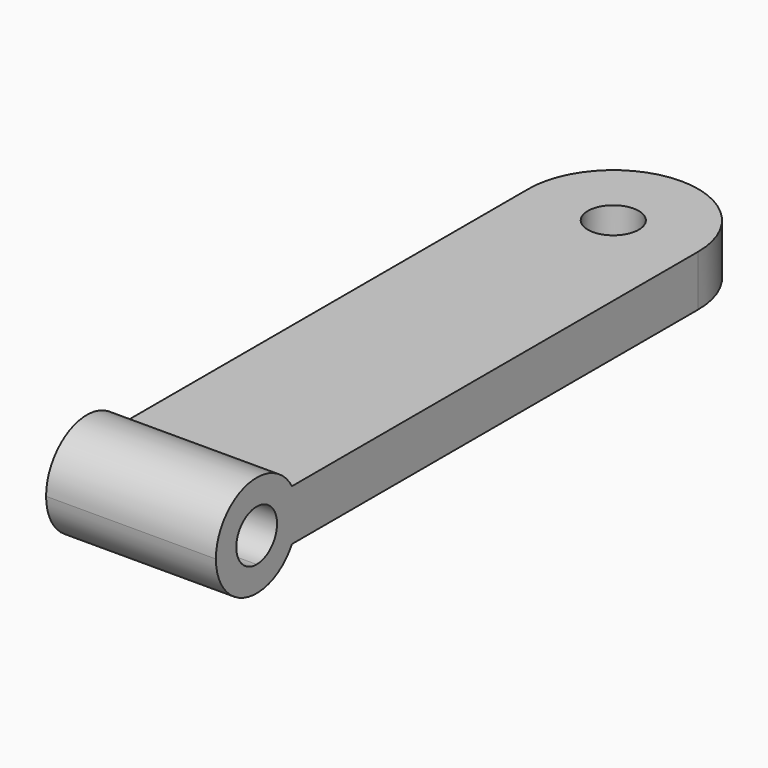
from build123d import *

# Parameters (mm, degrees)
F0_R     = 1.5
F1_DEPTH = 3
F3_DEPTH = 10
F4_DEPTH = 10.001


with BuildPart() as f1:
    # F0 (on Top) → F1 (new body)
    with BuildSketch(Plane.XY):
        with BuildLine():
            Line((-5, -17.5), (5, -17.5))
            Line((5, -17.5), (5, 17.5))
            ThreePointArc((5, 17.5), (0, 22.5), (-5, 17.5))
            Line((-5, 17.5), (-5, -17.5))
        make_face()
        with Locations((0, 17.5)):
            Circle(F0_R, mode=Mode.SUBTRACT)
    extrude(amount=F1_DEPTH)

    # F2 (on face) → F3 (join, through all)
    with BuildSketch(Plane(origin=(-5, 0, 0), x_dir=(0, -1, 0), z_dir=(-1, 0, 0))):
        with BuildLine():
            ThreePointArc((15, 3), (16.0606601718, 2.5606601718), (16.5, 1.5))
            ThreePointArc((16.5, 1.5), (16.0606601718, 0.4393398282), (15, 0))
            Line((15, 0), (17.5, 0))
            Line((17.5, 0), (17.5, 3))
            Line((17.5, 3), (15, 3))
        make_face()
        with BuildLine():
            Line((12.4019237886, 3), (15, 3))
            Line((15, 3), (17.5, 3))
            Line((17.5, 3), (17.5, 0))
            Line((17.5, 0), (15, 0))
            Line((15, 0), (12.4019237886, 0))
            ThreePointArc((12.4019237886, 0), (15.7764571353, -1.3977774789), (18, 1.5))
            ThreePointArc((18, 1.5), (15.7764571353, 4.3977774789), (12.4019237886, 3))
        make_face()
    extrude(amount=-F3_DEPTH)

    # F2 (on face) → F4 (cut, through all)
    with BuildSketch(Plane(origin=(-5, 0, 0), x_dir=(0, -1, 0), z_dir=(-1, 0, 0))):
        with BuildLine():
            ThreePointArc((15, 0), (16.0606601718, 0.4393398282), (16.5, 1.5))
            ThreePointArc((16.5, 1.5), (16.0606601718, 2.5606601718), (15, 3))
            ThreePointArc((15, 3), (13.5, 1.5), (15, 0))
        make_face()
    extrude(amount=-F4_DEPTH, mode=Mode.SUBTRACT)


solid = f1.part
